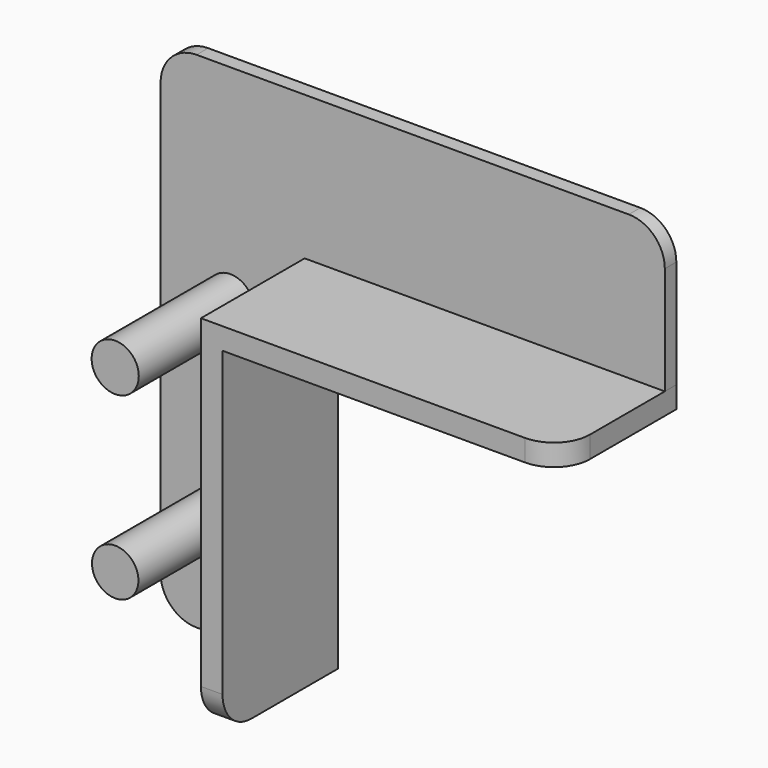
from build123d import *

# Parameters (mm, degrees)
F1_DEPTH = 10
F3_DEPTH = 2
F4_R     = 3.2736436262
F4_R_2   = 3.2241635896
F5_DEPTH = 20
F6_R     = 5
F6_2_R   = 5


# Not quite as in the source:
# - the program builds the solid bodies; features that only make, move or delete a surface that nothing else refers to are left out


with BuildPart() as f1:
    # F0 (on Front) → F1 (new body, symmetric)
    with BuildSketch(Plane.XZ):
        Polygon((25, 22), (25, 25), (-25, 25), (-25, -25), (-22, -25), (-22, -22), (-22, 22), (22, 22), align=None)
    extrude(amount=F1_DEPTH, both=True)

    # F6
    f6_edges = [f1.edges().sort_by_distance(p)[0] for p in [
        (25, -10, 23.5),
        (-23.5, -10, -25),
    ]]
    fillet(f6_edges, radius=F6_R)


with BuildPart() as f3:
    # F2 (on face) → F3 (new body)
    with BuildSketch(Plane(origin=(0, 10, 0), x_dir=(-1, 0, 0), z_dir=(0, 1, 0))):
        Polygon((-25, 45), (-25, 25), (25, 25), (25, -25), (45, -25), (45, 45), align=None)
    extrude(amount=-F3_DEPTH)

    # F4 (on face) → F5 (join)
    with BuildSketch(Plane.XZ.offset(-8)):
        with Locations((-35.3017263114, 16.4514879785)):
            Circle(F4_R)
        with Locations((-35.3017263114, -8.5485120215)):
            Circle(F4_R_2)
    extrude(amount=F5_DEPTH)

    # F6#2
    f6_2_edges = [f3.edges().sort_by_distance(p)[0] for p in [
        (25, 9, 45),
        (-45, 9, -25),
        (-45, 9, 45),
    ]]
    fillet(f6_2_edges, radius=F6_2_R)


solid = Compound([f1.part, f3.part])
